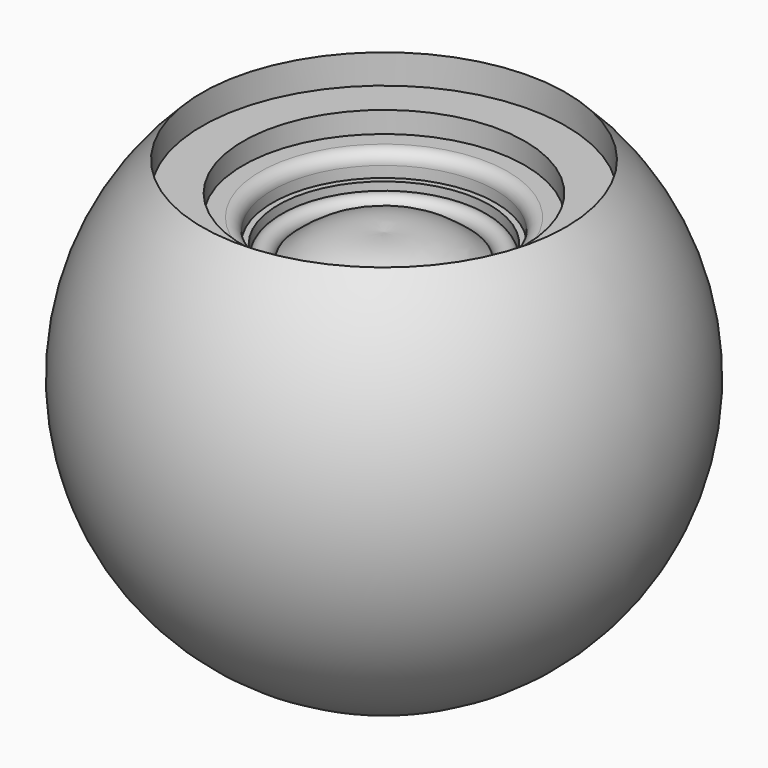
from build123d import *


# Not quite as in the source:
# - the program builds the solid bodies; features that only make, move or delete a surface that nothing else refers to are left out


with BuildPart() as f1:
    # F0 (on Front) → F1 (revolve)
    with BuildSketch(Plane.XZ):
        with BuildLine():
            Line((31, 29.0400044304), (24, 29.0400044304))
            Line((24, 29.0400044304), (24, 9.0400044304))
            ThreePointArc((24, 9.0400044304), (19.6066017178, -1.5665972874), (9, -5.9599955696))
            Line((9, -5.9599955696), (0, -5.9599955696))
            Line((0, -5.9599955696), (0, -7.9599955696))
            Line((0, -7.9599955696), (9, -7.9599955696))
            ThreePointArc((9, -7.9599955696), (21.0208152802, -2.9808108498), (26, 9.0400044304))
            Line((26, 9.0400044304), (26, 27.0400044304))
            Line((26, 27.0400044304), (34.5349993492, 27.0400044304))
            ThreePointArc((34.5349993492, 27.0400044304), (38.4097484566, -17.9101031612), (0, -41.5790084302))
            Line((0, -41.5790084302), (0, -43.5790084302))
            ThreePointArc((0, -43.5790084302), (41.7902834324, -15.2694910667), (31, 34.0400044304))
            Line((31, 34.0400044304), (31, 29.0400044304))
        make_face()
    revolve(axis=Axis((0, 0, -1.3016499579), (0, 0, -1)))


with BuildPart() as f3:
    # F2 (on Front) → F3 (revolve)
    with BuildSketch(Plane.XZ):
        with BuildLine():
            Line((29, 19.4262499511), (29, 25.4262499511))
            Line((29, 25.4262499511), (21.1, 25.4262499511))
            ThreePointArc((21.1, 25.4262499511), (19.6150757595, 24.8111741916), (19, 23.3262499511))
            Line((19, 23.3262499511), (19, 21.4378833771))
            Line((19, 21.4378833771), (18, 21.4378833771))
            Line((18, 21.4378833771), (18, 18.9806893468))
            ThreePointArc((18, 18.9806893468), (16.25, 20.7306893468), (14.5, 18.9806893468))
            add(Edge.make_bspline(
                [(14.5, 18.9806893468), (9.9864555523, 23.0175070465), (5.1598250866, 23.8073188812), (0, 23.1930203736)],
                knots=[0, 0, 0, 0, 15.0994613374, 15.0994613374, 15.0994613374, 15.0994613374], degree=3))
            Line((0, 23.1930203736), (0, 10.3049101308))
            Line((0, 10.3049101308), (20.4229932278, 10.3049101308))
            Line((20.4229932278, 10.3049101308), (20.4229932278, 19.4262499511))
            Line((20.4229932278, 19.4262499511), (29, 19.4262499511))
        make_face()
    revolve(axis=Axis((0, 0, 19.5949868066), (0, 0, -1)))


solid = Compound([f1.part, f3.part])
